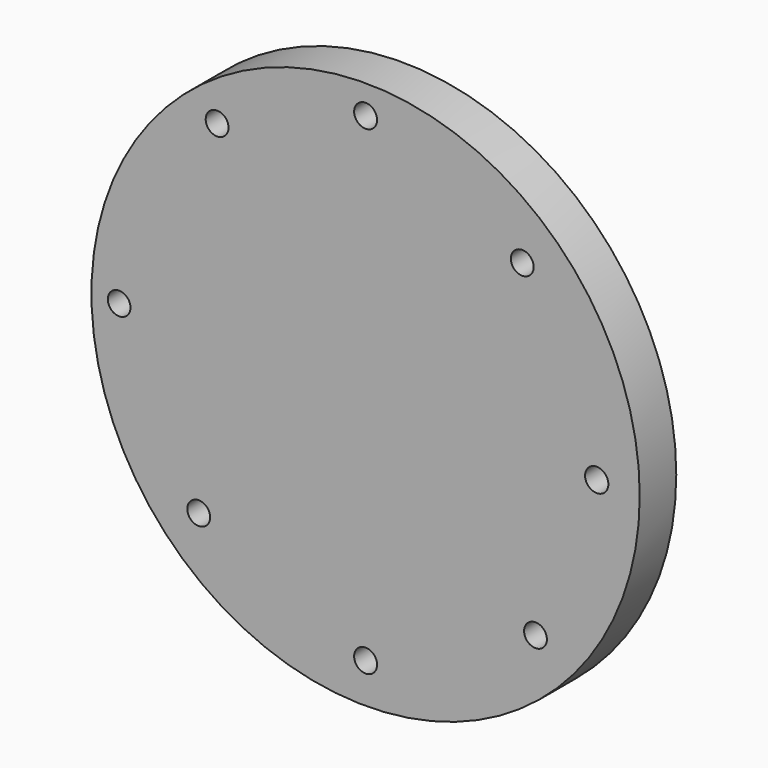
from build123d import *

# Parameters (mm, degrees)
F0_R     = 76.2210632732
F1_DEPTH = 12.7
F2_R     = 3.1879491609
F2_R_2   = 3.1879465914
F2_R_3   = 3.2380529084
F2_R_4   = 3.1498446293
F2_R_5   = 3.1721232023
F2_R_6   = 3.1721218695
F2_R_7   = 3.1721255347
F2_R_8   = 3.1721262011
F3_DEPTH = 25.4


# Not quite as in the source:
# - a length typed as a fraction of an inch, garbled in the dataset ("3 / 203.2 mm" for 3/8 in), is restored


with BuildPart() as f1:
    # F0 (on Front) → F1 (new body)
    with BuildSketch(Plane.XZ):
        Circle(F0_R)
    extrude(amount=F1_DEPTH)

    # F2 (on Front) → F3 (cut)
    with BuildSketch(Plane.XZ):
        with Locations((0, 68.2354792953)):
            Circle(F2_R)
        with Locations((0, -65.1145204902)):
            Circle(F2_R_2)
        with Locations((64.2633512616, 0)):
            Circle(F2_R_3)
        with Locations((-68.519204855, 0)):
            Circle(F2_R_4)
        with Locations((-41.2817560136, 52.9144145548)):
            Circle(F2_R_5)
        with Locations((47.2399480641, -43.5515418649)):
            Circle(F2_R_6)
        with Locations((-46.3887788355, -44.118989259)):
            Circle(F2_R_7)
        with Locations((43.5515418649, 46.3887788355)):
            Circle(F2_R_8)
    extrude(amount=F3_DEPTH, mode=Mode.SUBTRACT)


solid = f1.part
